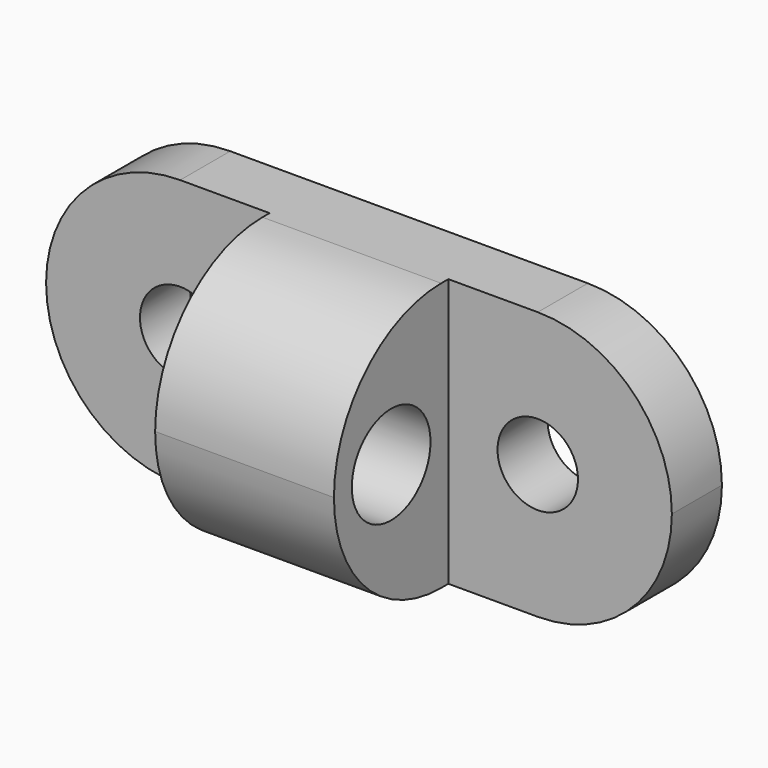
from build123d import *

# Parameters (mm, degrees)
F0_W      = 3556
F0_H      = 1524
F1_DEPTH  = 1168.4
F2_W      = 1505.427623216
F2_H      = 2067.9539636784
F3_DEPTH  = 812.8
F4_W      = 1708.8952731906
F4_H      = 3574.3826215129
F5_DEPTH  = 812.8
F6_R      = 761.99999
F7_R      = 761.99999
F9_R      = 228.6
F10_DEPTH = 355.601
F8_R      = 228.6
F11_DEPTH = 355.601
F12_R     = 279.4
F13_DEPTH = 2286.001


# Not quite as in the source:
# - a fillet or chamfer is up to 0.001 mm smaller than in the source, because OpenCascade refuses the exact size


with BuildPart() as f1:
    # F0 (on Front) → F1 (new body)
    with BuildSketch(Plane.XZ):
        with Locations((10.5376988649, -257.9351535461)):
            Rectangle(F0_W, F0_H)
    extrude(amount=F1_DEPTH)

    # F2 (on face) → F3 (cut)
    with BuildSketch(Plane.XZ.offset(1168.4)):
        with Locations((-1250.1761127431, -206.1067819595)):
            Rectangle(F2_W, F2_H)
    extrude(amount=-F3_DEPTH, mode=Mode.SUBTRACT)

    # F4 (on face) → F5 (cut)
    with BuildSketch(Plane.XZ.offset(1168.4)):
        with Locations((1372.9853354602, -353.8175821304)):
            Rectangle(F4_W, F4_H)
    extrude(amount=-F5_DEPTH, mode=Mode.SUBTRACT)

    # F6 (radius 762 in the source; OpenCascade refuses exactly that, so slightly less here)
    f6_edges = [f1.edges().sort_by_distance(p)[0] for p in [
        (10.537699, -1168.4, 504.064846),
        (10.537699, -1168.4, -1019.935154),
    ]]
    fillet(f6_edges, radius=F6_R)

    # F7 (radius 762 in the source; OpenCascade refuses exactly that, so slightly less here)
    f7_edges = [f1.edges().sort_by_distance(p)[0] for p in [
        (1788.537699, -177.8, -1019.935154),
        (1788.537699, -177.8, 504.064846),
        (-1767.462301, -177.8, 504.064846),
        (-1767.462301, -177.8, -1019.935154),
    ]]
    fillet(f7_edges, radius=F7_R)

    # F9 (on face) → F10 (cut, through all)
    with BuildSketch(Plane.XZ.offset(355.6)):
        with Locations((1026.5376988649, -257.9351535461)):
            Circle(F9_R)
    extrude(amount=-F10_DEPTH, mode=Mode.SUBTRACT)

    # F8 (on face) → F11 (cut, through all)
    with BuildSketch(Plane.XZ.offset(355.6)):
        with Locations((-1005.4623011351, -257.9351535461)):
            Circle(F8_R)
    extrude(amount=-F11_DEPTH, mode=Mode.SUBTRACT)

    # F12 (on face) → F13 (cut, through all)
    with BuildSketch(Plane.YZ.offset(518.5376988649)):
        with Locations((-762, -257.9351535461)):
            Circle(F12_R)
    extrude(amount=-F13_DEPTH, mode=Mode.SUBTRACT)


solid = f1.part
